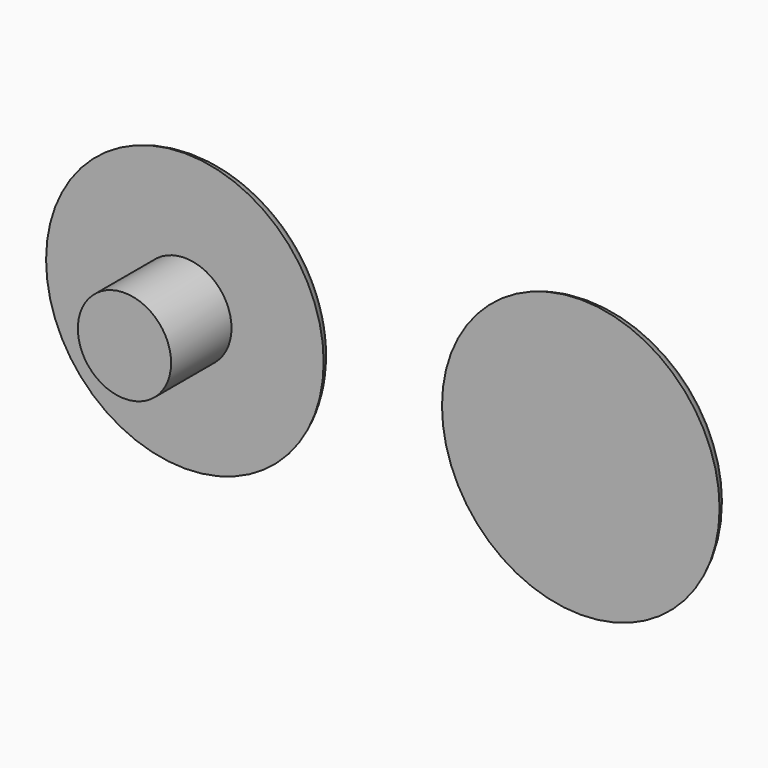
from build123d import *

# Parameters (mm, degrees)
F0_R     = 4.2
F1_DEPTH = 6.8
F3_R     = 12.5
F3_R_2   = 4.2
F4_DEPTH = 2
F6_R     = 12.5
F7_DEPTH = 2


# Not quite as in the source:
# - a fillet or chamfer that OpenCascade refuses, or shapes differently, is made with other operations: its cross-section is extruded or revolved along the edge and cut away or added


with BuildPart() as f1:
    # F0 (on Front) → F1 (new body)
    with BuildSketch(Plane.XZ):
        Circle(F0_R)
    extrude(amount=F1_DEPTH)


with BuildPart() as f1_1:
    # F2: moved
    add(f1.part.moved(Location((0, -2, 0))))

    # F3 (on face) → F4 (join)
    with BuildSketch(Plane(origin=(0, -2, 0), x_dir=(-1, 0, 0), z_dir=(0, 1, 0))):
        Circle(F3_R)
        Circle(F3_R_2, mode=Mode.SUBTRACT)
        Circle(F3_R_2)
    extrude(amount=F4_DEPTH)

    # F5: fillet of radius 3 on 1 edges, made by hand

    # F5_s1 → F5_t2 (revolve, cut)
    with BuildSketch(Plane.XY):
        with BuildLine():
            ThreePointArc((-12.5, -2), (-11.4036236828, -0.5505102572), (-9.6715728753, 0))
            Line((-9.6715728753, 0), (-12.5, 0))
            Line((-12.5, 0), (-12.5, -2))
        make_face()
    revolve(axis=Axis((0, 0, 0), (0, 1, 0)), mode=Mode.SUBTRACT)


with BuildPart() as f7:
    # F6 (on Front) → F7 (new body)
    with BuildSketch(Plane.XZ):
        with Locations((35.6552414596, 0)):
            Circle(F6_R)
    extrude(amount=F7_DEPTH)

    # F8: fillet of radius 3 on 1 edges, made by hand

    # F8_s1 → F8_t2 (revolve, cut)
    with BuildSketch(Plane.XY):
        with BuildLine():
            ThreePointArc((48.1552414596, -2), (47.0588651424, -0.5505102572), (45.3268143349, 0))
            Line((45.3268143349, 0), (48.1552414596, 0))
            Line((48.1552414596, 0), (48.1552414596, -2))
        make_face()
    revolve(axis=Axis((35.6552414596, 0, 0), (0, -1, 0)), mode=Mode.SUBTRACT)


solid = Compound([f1_1.part, f7.part])
